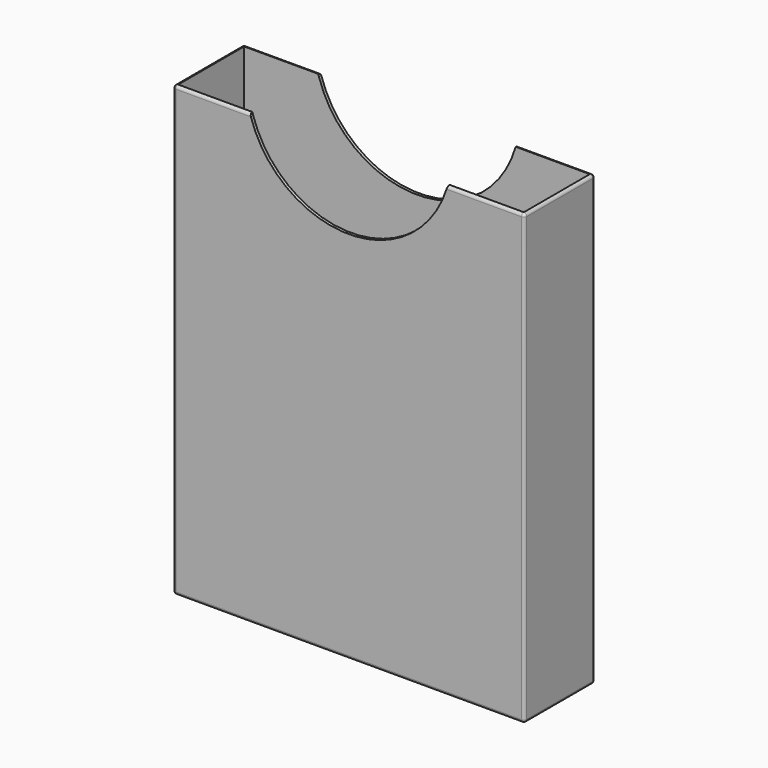
from build123d import *

# Parameters (mm, degrees)
F0_W     = 121.5
F0_H     = 30.5
F0_W_2   = 119.5
F0_H_2   = 28.5
F1_DEPTH = 155
F2_DEPTH = 1
F3_R     = 0.99999
F5_DEPTH = 30.5


# Not quite as in the source:
# - a fillet or chamfer is up to 0.001 mm smaller than in the source, because OpenCascade refuses the exact size


with BuildPart() as f1:
    # F0 (on Top) → F1 (new body)
    with BuildSketch(Plane.XY):
        with Locations((7.2500004172, -0.2499995828)):
            Rectangle(F0_W, F0_H)
        with Locations((7.2500004172, -0.2499995828)):
            Rectangle(F0_W_2, F0_H_2, mode=Mode.SUBTRACT)
    extrude(amount=F1_DEPTH)

    # F0 (on Top) → F2 (join)
    with BuildSketch(Plane.XY):
        with Locations((7.2500004172, -0.2499995828)):
            Rectangle(F0_W_2, F0_H_2)
    extrude(amount=F2_DEPTH)

    # F3 (radius 1 in the source; OpenCascade refuses exactly that, so slightly less here)
    f3_edges = [f1.edges().sort_by_distance(p)[0] for p in [
        (68, -15.5, 77.5),
        (68, 15, 77.5),
        (68, -0.25, 0),
        (7.25, 15, 0),
        (7.25, -15.5, 0),
        (-53.5, -0.25, 0),
        (-53.5, -15.5, 77.5),
        (-53.5, 15, 77.5),
        (7.25, -15.5, 155),
        (-53.5, -0.25, 155),
        (7.25, 15, 155),
        (68, -0.25, 155),
    ]]
    fillet(f3_edges, radius=F3_R)

    # F4 (on face) → F5 (cut, through all)
    with BuildSketch(Plane(origin=(0, 15.0000004172, 0), x_dir=(-1, 0, 0), z_dir=(0, 1, 0))):
        with BuildLine():
            ThreePointArc((26.5693810998, 154.00001), (27.8320116519, 159.3416659555), (28.2562680656, 164.8140996695))
            ThreePointArc((28.2562680656, 164.8140996695), (-12.7224341312, 199.8961117386), (-41.0693819342, 154.00001))
            Line((-41.0693819342, 154.00001), (-7.2500004172, 154.00001))
            Line((-7.2500004172, 154.00001), (26.5693810998, 154.00001))
        make_face()
        with BuildLine():
            Line((-7.2500004172, 154.00001), (-41.0693819342, 154.00001))
            ThreePointArc((-41.0693819342, 154.00001), (-7.2500004172, 129.3078311867), (26.5693810998, 154.00001))
            Line((26.5693810998, 154.00001), (-7.2500004172, 154.00001))
        make_face()
    extrude(amount=-F5_DEPTH, mode=Mode.SUBTRACT)


solid = f1.part
